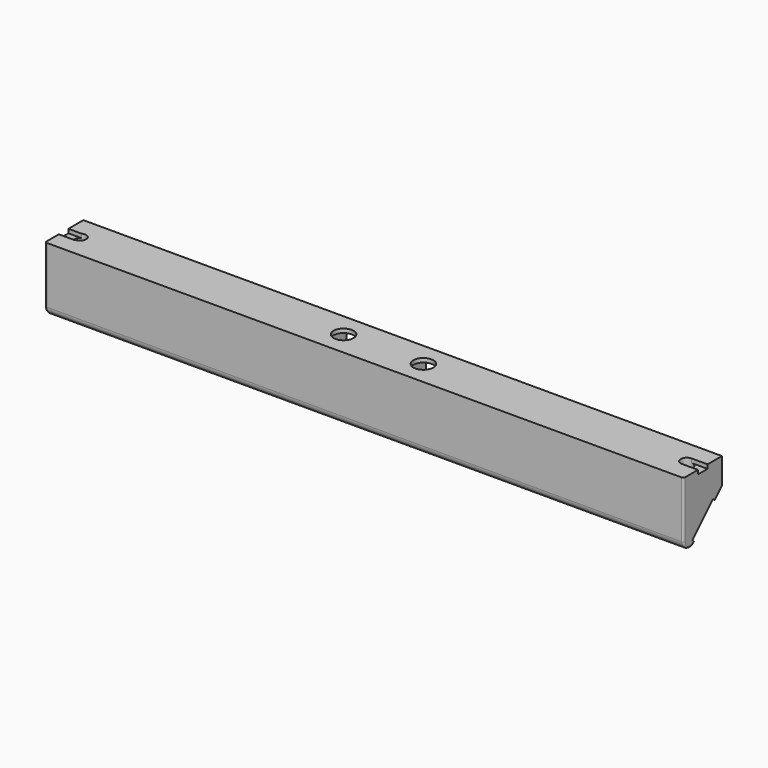
from build123d import *

# Parameters (mm, degrees)
F1_DEPTH = 160
F3_D     = 5
F3_DEPTH = 5
F3_TIP   = 1.5021515476
F4_W     = 8.2
F4_H     = 5.2
F5_DEPTH = 11
F7_D     = 3
F6_W     = 4
F6_H     = 3
F8_DEPTH = 1
F9_R     = 2
F10_R    = 0.5


# Not quite as in the source:
# - a feature names something its author has since deleted; it is built from what else it names


with BuildPart() as f1:
    # F0 (on Right) → F1 (new body)
    with BuildSketch(Plane.YZ):
        Polygon((9.9597979746, -9.0402020254), (12, -7), (12, 0), (0, 0), (0, -6.5), (0, -19), (3.4544155877, -15.5455844123), (2.7473088065, -14.8384776311), (9.2526911935, -8.3330952442), align=None)
    extrude(amount=F1_DEPTH)

    # F3
    with Locations(Plane.XY):
        with Locations((90, 6), (70, 6)):
            Hole(F3_D / 2, depth=F3_DEPTH)
            with Locations((0, 0, -(F3_DEPTH + F3_TIP / 2))):  # 118° drill point
                Cone(0, F3_D / 2, F3_TIP, mode=Mode.SUBTRACT)

    # F4 (on face) → F5 (cut)
    with BuildSketch(Plane(origin=(0, 12, 0), x_dir=(-1, 0, 0), z_dir=(0, 1, 0))):
        with Locations((-90, -3.6)):
            Rectangle(F4_W, F4_H)
        with Locations((-70, -3.6)):
            Rectangle(F4_W, F4_H)
    extrude(amount=-F5_DEPTH, mode=Mode.SUBTRACT)

    # F7 (through all)
    with Locations(Plane.XY):
        with Locations((4, 6), (156, 6)):
            Hole(F7_D / 2)

    # F6 (on Top) → F8 (cut)
    with BuildSketch(Plane.XY):
        with Locations((158, 6)):
            Rectangle(F6_W, F6_H)
        with Locations((2, 5.8232012801)):
            Rectangle(F6_W, F6_H)
    extrude(amount=-F8_DEPTH, mode=Mode.SUBTRACT)

    # F9
    f9_edges = [f1.edges().sort_by_distance(p)[0] for p in [
        (80, 0, -19),
    ]]
    fillet(f9_edges, radius=F9_R)

    # F10
    f10_edges = [f1.edges().sort_by_distance(p)[0] for p in [
        (160, 10.979899, -8.020101),
        (0, 10.979899, -8.020101),
        (160, 3.434315, -15.565685),
        (0, 3.434315, -15.565685),
        (0, 1.234633, -16.019332),
        (0, 0, -7.085786),
        (160, 1.234633, -16.019332),
        (160, 0, -7.085786),
        (80, 9.959798, -9.040202),
        (80, 12, -7),
    ]]
    fillet(f10_edges, radius=F10_R)


solid = f1.part
